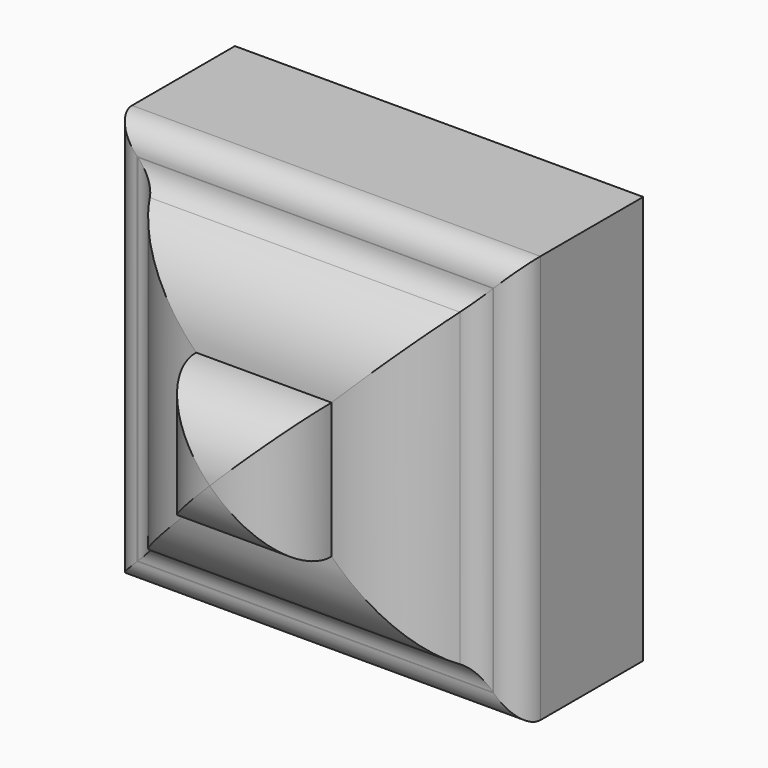
from build123d import *

# Parameters (mm, degrees)
F0_W        = 0.95
F0_H        = 0.95
F1_DEPTH    = 0.719
F2_W        = 0.75
F2_H        = 0.75
F3_DEPTH    = 0.3
F4_T1_DEPTH = 3.6740515173
F4_T3_DEPTH = 3.6740515173
F5_W        = 0.3151896965
F5_H        = 0.3151896965
F6_DEPTH    = 0.315
F7_R        = 0.314196
F8_R        = 0.1207106781


# Not quite as in the source:
# - a fillet or chamfer that OpenCascade refuses, or shapes differently, is made with other operations: its cross-section is extruded or revolved along the edge and cut away or added
# - a fillet or chamfer is up to 0.001 mm smaller than in the source, because OpenCascade refuses the exact size


with BuildPart() as f1:
    # F0 (on Front) → F1 (new body)
    with BuildSketch(Plane.XZ):
        Polygon((0, 0.95), (0, 0), (-0.95, 0), (-0.95, -0.95), (0, -0.95), (0.95, -0.95), (0.95, 0), (0.95, 0.95), align=None)
        with Locations((-0.475, 0.475)):
            Rectangle(F0_W, F0_H)
    extrude(amount=F1_DEPTH)

    # F2 (on face) → F3 (join)
    with BuildSketch(Plane.XZ.offset(0.719)):
        Polygon((0, 0.75), (0, 0), (-0.75, 0), (-0.75, -0.75), (0, -0.75), (0.75, -0.75), (0.75, 0), (0.75, 0.75), align=None)
        with Locations((-0.375, 0.375)):
            Rectangle(F2_W, F2_H)
    extrude(amount=F3_DEPTH)

    # F4: fillet of radius 0.4651 on 4 edges, made by hand

    # F4_s2 → F4_t1 (cut)
    with BuildSketch(Plane.YZ.offset(-1.8370257587)):
        with BuildLine():
            ThreePointArc((-0.719, -0.75), (-0.9367224262, -0.579320346), (-1.019, -0.3151896965))
            Line((-1.019, -0.3151896965), (-1.019, -0.75))
            Line((-1.019, -0.75), (-0.719, -0.75))
        make_face()
        with BuildLine():
            ThreePointArc((-0.719, 0.75), (-0.9367224262, 0.579320346), (-1.019, 0.3151896965))
            Line((-1.019, 0.3151896965), (-1.019, 0.75))
            Line((-1.019, 0.75), (-0.719, 0.75))
        make_face()
    extrude(amount=F4_T1_DEPTH, mode=Mode.SUBTRACT)

    # F4_s4 → F4_t3 (cut)
    with BuildSketch(Plane.XY.offset(-1.8370257587)):
        with BuildLine():
            ThreePointArc((0.75, -0.719), (0.579320346, -0.9367224262), (0.3151896965, -1.019))
            Line((0.3151896965, -1.019), (0.75, -1.019))
            Line((0.75, -1.019), (0.75, -0.719))
        make_face()
        with BuildLine():
            ThreePointArc((-0.75, -0.719), (-0.579320346, -0.9367224262), (-0.3151896965, -1.019))
            Line((-0.3151896965, -1.019), (-0.75, -1.019))
            Line((-0.75, -1.019), (-0.75, -0.719))
        make_face()
    extrude(amount=F4_T3_DEPTH, mode=Mode.SUBTRACT)

    # F5 (on face) → F6 (join)
    with BuildSketch(Plane.XZ.offset(1.019)):
        with Locations((-0.1575948483, 0.1575948483)):
            Rectangle(F5_W, F5_H)
        Polygon((0.3151896965, 0.3151896965), (0, 0.3151896965), (0, 0), (-0.3151896965, 0), (-0.3151896965, -0.3151896965), (0, -0.3151896965), (0.3151896965, -0.3151896965), (0.3151896965, 0), align=None)
    extrude(amount=F6_DEPTH)

    # F7 (radius 0.315196 in the source; OpenCascade refuses exactly that, so slightly less here)
    f7_edges = [f1.edges().sort_by_distance(p)[0] for p in [
        (-0.31519, -1.334, 0),
        (0, -1.334, -0.31519),
        (0.31519, -1.334, 0),
        (0, -1.334, 0.31519),
    ]]
    fillet(f7_edges, radius=F7_R)

    # F8
    f8_edges = [f1.edges().sort_by_distance(p)[0] for p in [
        (-0.95, -0.719, 0),
        (0, -0.719, -0.95),
        (0.95, -0.719, 0),
        (0, -0.719, 0.95),
        (-0.75, -0.719, 0),
        (0, -0.719, 0.75),
        (0.75, -0.719, 0),
        (0, -0.719, -0.75),
    ]]
    fillet(f8_edges, radius=F8_R)


solid = f1.part
